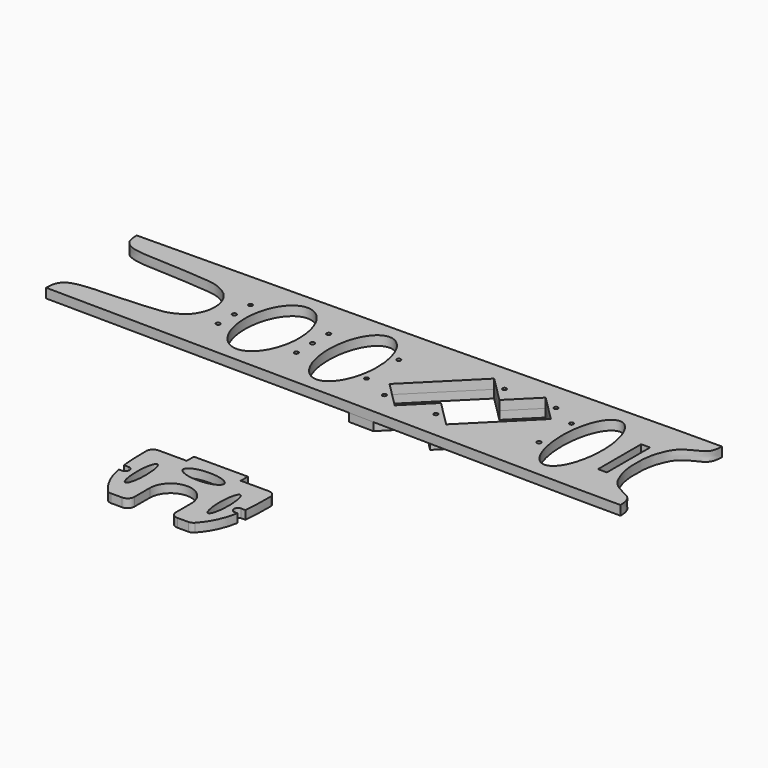
from build123d import *

# Parameters (mm, degrees)
F1_R     = 0.75
F1_W     = 3.3
F1_H     = 20
F2_DEPTH = 3.5
F3_R     = 0.75
F4_DEPTH = 3
F6_DEPTH = 3.2


# Not quite as in the source:
# - the dataset's text gives a spline's control points without its knots; the knots are read off the source's solid


with BuildPart() as f2:
    # F1 (on Top) → F2 (new body)
    with BuildSketch(Plane.XY):
        with BuildLine():
            add(Edge.make_bspline(
                [(-109.25, -3.3), (-82.9141073212, -2.8646297059), (-1.270729355, -2.3674163572), (32.7413898255, -1.6067550163), (59.4534914207, -1.377915026), (93.8122415195, -0.6959335272), (105.75, -0.8)],
                knots=[0, 0, 0, 0, 0.3675872258, 0.5786163549, 0.7605624284, 1, 1, 1, 1], degree=3))
            add(Edge.make_bspline(
                [(-109.25, -3.3), (-109.25, -5.8667144649), (-108.3286389403, -8.9811572378), (-103.1641587025, -11.1743671014), (-92.2247356374, -11.4488954751), (-83.2931944213, -11.9447685478), (-75.4315010969, -12.5391153919), (-71.8862448572, -13.0825399903), (-68.7783080633, -14.6141399054), (-66.2508920463, -16.4090381884), (-64.498047697, -19.1911246901), (-63.5718011871, -22.1286780395), (-63.5074121734, -23.6215211632), (-63.5074121734, -24.3)],
                knots=[0, 0, 0, 0, 0.0969821928, 0.1882524756, 0.3249155201, 0.4529640738, 0.567181229, 0.6449292481, 0.720249404, 0.7928137824, 0.8674151127, 0.9397252918, 1, 1, 1, 1], degree=3))
            add(Edge.make_bspline(
                [(-109.25, -45.3), (-109.25, -42.7332855351), (-108.3286389403, -39.6188427622), (-103.1641587025, -37.4256328986), (-92.2247356374, -37.1511045249), (-83.2931944213, -36.6552314522), (-75.4315010969, -36.0608846081), (-71.8862448572, -35.5174600097), (-68.7783080633, -33.9858600946), (-66.2508920463, -32.1909618116), (-64.498047697, -29.4088753099), (-63.5718011871, -26.4713219605), (-63.5074121734, -24.9784788368), (-63.5074121734, -24.3)],
                knots=[0, 0, 0, 0, 0.0969821928, 0.1882524756, 0.3249155201, 0.4529640738, 0.567181229, 0.6449292481, 0.720249404, 0.7928137824, 0.8674151127, 0.9397252918, 1, 1, 1, 1], degree=3))
            add(Edge.make_bspline(
                [(-109.25, -45.3), (-82.9141073212, -45.7353702941), (-1.270729355, -46.2325836428), (32.7413898255, -46.9932449837), (59.4534914207, -47.222084974), (93.8122415195, -47.9040664728), (105.75, -47.8)],
                knots=[0, 0, 0, 0, 0.3675872258, 0.5786163549, 0.7605624284, 1, 1, 1, 1], degree=3))
            add(Edge.make_bspline(
                [(105.75, -47.8), (105.75, -45.9220040834), (105.1286084932, -43.3378264927), (103.0015043689, -41.7930717229), (99.9244448741, -40.4874921286), (97.2696844232, -38.7008537465), (95.7496091876, -36.9007576711), (94.4789561408, -34.0717508148), (93.5187012908, -31.452382061), (92.9895349369, -28.4123411906), (92.8294994282, -26.216512958), (92.8608642426, -24.9274592576), (92.8608642426, -24.3)],
                knots=[0, 0, 0, 0, 0.1253807055, 0.2171241486, 0.325926749, 0.4317756476, 0.5223605214, 0.6256285419, 0.7263803974, 0.8302306108, 0.9184940732, 1, 1, 1, 1], degree=3))
            add(Edge.make_bspline(
                [(105.75, -0.8), (105.75, -2.6779959166), (105.1286084932, -5.2621735073), (103.0015043689, -6.8069282771), (99.9244448741, -8.1125078714), (97.2696844232, -9.8991462535), (95.7496091876, -11.6992423289), (94.4789561408, -14.5282491852), (93.5187012908, -17.147617939), (92.9895349369, -20.1876588094), (92.8294994282, -22.383487042), (92.8608642426, -23.6725407424), (92.8608642426, -24.3)],
                knots=[0, 0, 0, 0, 0.1253807055, 0.2171241486, 0.325926749, 0.4317756476, 0.5223605214, 0.6256285419, 0.7263803974, 0.8302306108, 0.9184940732, 1, 1, 1, 1], degree=3))
        make_face()
        with Locations((-56.25, -31.8)):
            Circle(F1_R, mode=Mode.SUBTRACT)
        with Locations((-27.25, -31.8)):
            Circle(F1_R, mode=Mode.SUBTRACT)
        with Locations((9.2837482372, -36.6743686708)):
            Circle(F1_R, mode=Mode.SUBTRACT)
        with Locations((28.3756313292, -36.6743686708)):
            Circle(F1_R, mode=Mode.SUBTRACT)
        with Locations((-1.25, -31.8)):
            Circle(F1_R, mode=Mode.SUBTRACT)
        Polygon((27.668524548, -8.7436508139), (37.2144660941, -18.2895923599), (46.7604076401, -8.7436508139), (56.3063491861, -18.2895923599), (34.7395923599, -39.8563491861), (25.1936508139, -30.3104076401), (15.6477092679, -39.8563491861), (6.1017677219, -30.3104076401), align=None, mode=Mode.SUBTRACT)
        with Locations((62.75, -31.8)):
            Circle(F1_R, mode=Mode.SUBTRACT)
        with Locations((-56.25, -24.3)):
            Circle(F1_R, mode=Mode.SUBTRACT)
        with Locations((-56.25, -16.8)):
            Circle(F1_R, mode=Mode.SUBTRACT)
        with BuildLine():
            add(Edge.make_bspline(
                [(-32.25, -24.3), (-32.25, 4.2788383249), (-47.25, -10.0105808376), (-62.25, -24.3), (-47.25, -38.5894191624), (-32.25, -52.8788383249), (-32.25, -24.3)],
                knots=[4.7123889804, 4.7123889804, 4.7123889804, 6.8067840828, 6.8067840828, 8.9011791852, 8.9011791852, 10.9955742876, 10.9955742876, 10.9955742876], degree=2, weights=[1, 0.5, 1, 0.5, 1, 0.5, 1]))
        make_face(mode=Mode.SUBTRACT)
        with Locations((-27.25, -24.3)):
            Circle(F1_R, mode=Mode.SUBTRACT)
        with BuildLine():
            add(Edge.make_bspline(
                [(-3.25, -24.3), (-3.25, 5.1448637287), (-16.75, -9.5775681357), (-30.25, -24.3), (-16.75, -39.0224318643), (-3.25, -53.7448637287), (-3.25, -24.3)],
                knots=[4.7123889804, 4.7123889804, 4.7123889804, 6.8067840828, 6.8067840828, 8.9011791852, 8.9011791852, 10.9955742876, 10.9955742876, 10.9955742876], degree=2, weights=[1, 0.5, 1, 0.5, 1, 0.5, 1]))
        make_face(mode=Mode.SUBTRACT)
        with Locations((-27.25, -16.8)):
            Circle(F1_R, mode=Mode.SUBTRACT)
        with Locations((-1.25, -16.8)):
            Circle(F1_R, mode=Mode.SUBTRACT)
        with BuildLine():
            add(Edge.make_bspline(
                [(65.25, -24.3), (65.25, -54.6108891325), (76.5, -39.4554445662), (87.75, -24.3), (76.5, -9.1445554338), (65.25, 6.0108891325), (65.25, -24.3)],
                knots=[4.7123889804, 4.7123889804, 4.7123889804, 6.8067840828, 6.8067840828, 8.9011791852, 8.9011791852, 10.9955742876, 10.9955742876, 10.9955742876], degree=2, weights=[1, 0.5, 1, 0.5, 1, 0.5, 1]))
        make_face(mode=Mode.SUBTRACT)
        with Locations((88.25, -24.3)):
            Rectangle(F1_W, F1_H, mode=Mode.SUBTRACT)
        with Locations((62.75, -16.8)):
            Circle(F1_R, mode=Mode.SUBTRACT)
        with Locations((34.0324855787, -11.9256313292)):
            Circle(F1_R, mode=Mode.SUBTRACT)
        with Locations((53.1243686708, -11.9256313292)):
            Circle(F1_R, mode=Mode.SUBTRACT)
    extrude(amount=F2_DEPTH)


with BuildPart() as f4:
    # F3 (on Top) → F4 (new body)
    with BuildSketch(Plane.XY):
        with BuildLine():
            Line((4.1017677219, -28.067766953), (4.1017677219, -46.4727957152))
            add(Edge.make_bspline(
                [(4.1017677219, -46.4727957152), (7.4012846458, -46.5166519222), (10.390571843, -46.5605461481), (13.1430766754, -46.6036224657)],
                knots=[0.3930476629, 0.3930476629, 0.3930476629, 0.3930476629, 0.438949806, 0.438949806, 0.438949806, 0.438949806], degree=3))
            Line((13.1430766754, -46.6036224657), (23.7794396962, -35.9672594449))
            Line((23.7794396962, -35.9672594449), (33.3253812422, -45.5132009909))
            Line((33.3253812422, -45.5132009909), (58.3063491861, -20.532233047))
            Line((58.3063491861, -20.532233047), (58.3063491861, -1.3271105974))
            add(Edge.make_bspline(
                [(49.8186787246, -1.4427390423), (52.4549743932, -1.4093523966), (55.2567510716, -1.3720792198), (58.3063491861, -1.3271105974)],
                knots=[0.6970426117, 0.6970426117, 0.6970426117, 0.6970426117, 0.7502287702, 0.7502287702, 0.7502287702, 0.7502287702], degree=3))
            Line((49.8186787246, -1.4427390423), (38.6286818684, -12.6327358985))
            Line((38.6286818684, -12.6327358985), (29.0827403223, -3.0867943525))
            Line((29.0827403223, -3.0867943525), (4.1017677219, -28.067766953))
        make_face()
        with Locations((9.2837482372, -36.6743686708)):
            Circle(F3_R, mode=Mode.SUBTRACT)
        with Locations((28.3756313292, -36.6743686708)):
            Circle(F3_R, mode=Mode.SUBTRACT)
        Polygon((25.1936508139, -30.3104076401), (15.6477092679, -39.8563491861), (6.1017677219, -30.3104076401), (27.668524548, -8.7436508139), (37.2144660941, -18.2895923599), (46.7604076401, -8.7436508139), (56.3063491861, -18.2895923599), (34.7395923599, -39.8563491861), align=None, mode=Mode.SUBTRACT)
        with Locations((34.0324855787, -11.9256313292)):
            Circle(F3_R, mode=Mode.SUBTRACT)
        with Locations((53.1243686708, -11.9256313292)):
            Circle(F3_R, mode=Mode.SUBTRACT)
    extrude(amount=-F4_DEPTH)


with BuildPart() as f6:
    # F5 (on Top) → F6 (new body)
    with BuildSketch(Plane.XY):
        with BuildLine():
            Line((10.2102639527, -133.8083887326), (14.2814403178, -133.8083887326))
            ThreePointArc((14.2814403178, -133.8083887326), (15.2951808284, -133.5936305529), (16.1347540856, -132.9862528743))
            add(Edge.make_bspline(
                [(22.0313273632, -120.6645872098), (21.1393270069, -125.2375208096), (19.4259298183, -129.3509279716), (16.1347540856, -132.9862528743)],
                knots=[15.376290751, 15.376290751, 15.376290751, 15.376290751, 29.5355188595, 29.5355188595, 29.5355188595, 29.5355188595], degree=3))
            Line((22.0313273632, -120.6645872098), (20.9855914014, -120.6645872098))
            ThreePointArc((20.9855914014, -120.6645872098), (19.4855914014, -119.1645872098), (20.9855914014, -117.6645872098))
            Line((20.9855914014, -117.6645872098), (22.4987020439, -117.6645872098))
            add(Edge.make_bspline(
                [(22.9973170132, -106.6727097733), (22.9846616845, -110.5678046063), (22.9123126792, -114.2340662597), (22.4987020439, -117.6645872098)],
                knots=[2.1593949599, 2.1593949599, 2.1593949599, 2.1593949599, 12.3450034741, 12.3450034741, 12.3450034741, 12.3450034741], degree=3))
            ThreePointArc((22.9973170132, -106.6727097733), (22.2679665924, -104.8996943531), (20.4973302085, -104.1645872098))
            Line((20.4973302085, -104.1645872098), (10, -104.1645872098))
            Line((10, -104.1645872098), (10, -100.8418556213))
            Line((10, -100.8418556213), (-10, -100.8418556213))
            Line((-10, -100.8418556213), (-10, -104.1645872098))
            Line((-10, -104.1645872098), (-20.4973302085, -104.1645872098))
            ThreePointArc((-20.4973302085, -104.1645872098), (-22.2679665924, -104.8996943531), (-22.9973170132, -106.6727097733))
            add(Edge.make_bspline(
                [(-22.9973170132, -106.6727097733), (-22.9846616845, -110.5678046063), (-22.9123126792, -114.2340662597), (-22.4987020439, -117.6645872098)],
                knots=[2.1593949599, 2.1593949599, 2.1593949599, 2.1593949599, 12.3450034741, 12.3450034741, 12.3450034741, 12.3450034741], degree=3))
            Line((-22.4987020439, -117.6645872098), (-20.7743608055, -117.6645872098))
            ThreePointArc((-20.7743608055, -117.6645872098), (-19.2743608055, -119.1645872098), (-20.7743608055, -120.6645872098))
            Line((-20.7743608055, -120.6645872098), (-22.0313273632, -120.6645872098))
            add(Edge.make_bspline(
                [(-22.0313273632, -120.6645872098), (-21.1393270069, -125.2375208096), (-19.4259298183, -129.3509279716), (-16.1347540856, -132.9862528743)],
                knots=[15.376290751, 15.376290751, 15.376290751, 15.376290751, 29.5355188595, 29.5355188595, 29.5355188595, 29.5355188595], degree=3))
            ThreePointArc((-16.1347540856, -132.9862528743), (-15.2951808284, -133.5936305529), (-14.2814403178, -133.8083887326))
            Line((-14.2814403178, -133.8083887326), (-10.2102639527, -133.8083887326))
            ThreePointArc((-10.2102639527, -133.8083887326), (-8.4424969997, -133.0761556856), (-7.7102639527, -131.3083887326))
            Line((-7.7102639527, -131.3083887326), (-7.7102639527, -124.1645872098))
            ThreePointArc((-7.7102639527, -124.1645872098), (0, -116.4543232571), (7.7102639527, -124.1645872098))
            Line((7.7102639527, -124.1645872098), (7.7102639527, -131.3083887326))
            ThreePointArc((7.7102639527, -131.3083887326), (8.4424969997, -133.0761556856), (10.2102639527, -133.8083887326))
        make_face()
        with BuildLine():
            add(Edge.make_bspline(
                [(-15.3699557171, -111.120931636), (-18.3244764919, -111.120931636), (-16.8472161045, -122.2114543187), (-15.3699557171, -133.3019770014), (-13.8926953297, -122.2114543187), (-12.4154349423, -111.120931636), (-15.3699557171, -111.120931636)],
                knots=[0, 0, 0, 2.0943951024, 2.0943951024, 4.1887902048, 4.1887902048, 6.2831853072, 6.2831853072, 6.2831853072], degree=2, weights=[1, 0.5, 1, 0.5, 1, 0.5, 1]))
        make_face(mode=Mode.SUBTRACT)
        with BuildLine():
            add(Edge.make_bspline(
                [(15.3699557171, -111.120931636), (12.4154349423, -111.120931636), (13.8926953297, -122.2114543187), (15.3699557171, -133.3019770014), (16.8472161045, -122.2114543187), (18.3244764919, -111.120931636), (15.3699557171, -111.120931636)],
                knots=[0, 0, 0, 2.0943951024, 2.0943951024, 4.1887902048, 4.1887902048, 6.2831853072, 6.2831853072, 6.2831853072], degree=2, weights=[1, 0.5, 1, 0.5, 1, 0.5, 1]))
        make_face(mode=Mode.SUBTRACT)
        with BuildLine():
            add(Edge.make_bspline(
                [(7.5, -108.8378429413), (7.5, -103.8591164126), (-3.75, -106.3484796769), (-15, -108.8378429413), (-3.75, -111.3272062056), (7.5, -113.81656947), (7.5, -108.8378429413)],
                knots=[0, 0, 0, 2.0943951024, 2.0943951024, 4.1887902048, 4.1887902048, 6.2831853072, 6.2831853072, 6.2831853072], degree=2, weights=[1, 0.5, 1, 0.5, 1, 0.5, 1]))
        make_face(mode=Mode.SUBTRACT)
    extrude(amount=F6_DEPTH)


solid = Compound([f2.part, f4.part, f6.part])
